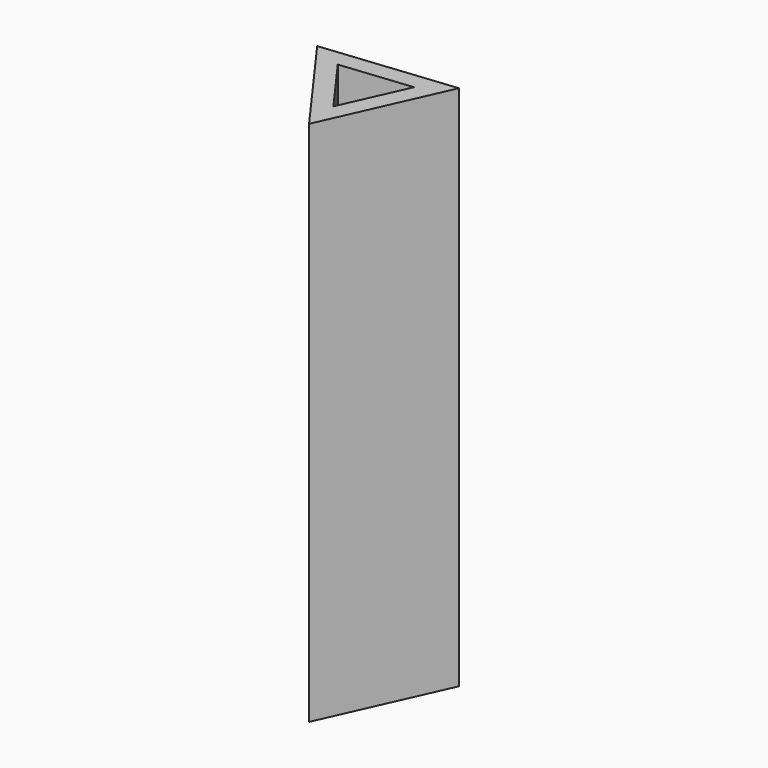
from build123d import *

# Parameters (mm, degrees)
F1_DEPTH = 304.8
F2_T     = -10.16


# Not quite as in the source:
# - a length typed as a fraction of an inch, garbled in the dataset ("3 / 203.2 mm" for 3/8 in), is restored


with BuildPart() as f1:
    # F0 (on Top) → F1 (new body)
    with BuildSketch(Plane.XY):
        Polygon((35.6380517451, 25.7955280584), (-40.1586084752, 17.9656941234), (4.5205567301, -43.7612221819), align=None)
    extrude(amount=F1_DEPTH)

    # F2
    f2_openings = [f1.faces().sort_by_distance(p)[0] for p in [
        (0, 0, 304.8),
    ]]
    offset(amount=F2_T, openings=f2_openings)


solid = f1.part
